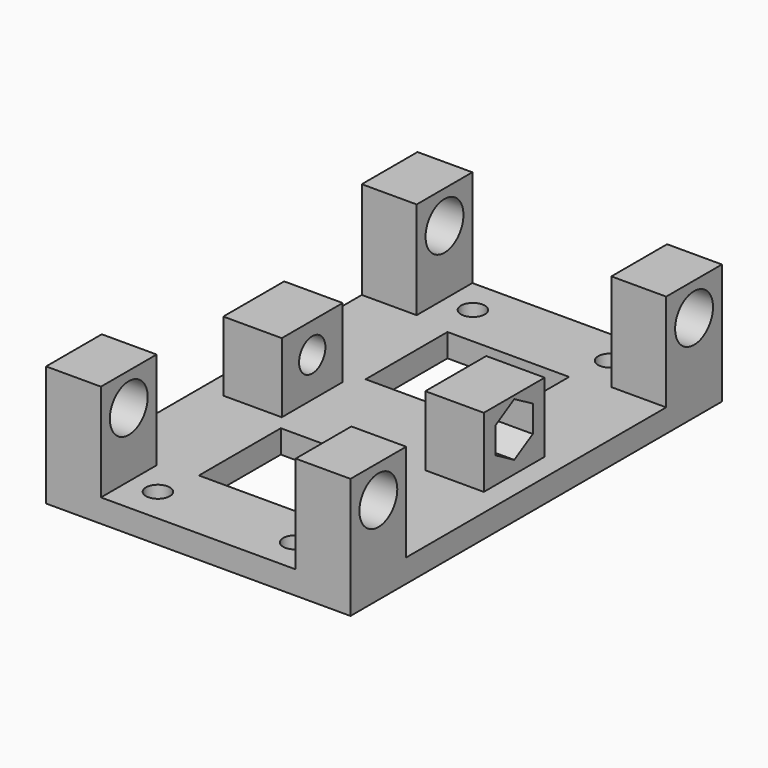
from build123d import *

# Parameters (mm, degrees)
F0_W      = 83.264
F0_H      = 127
F1_DEPTH  = 6.35
F2_W      = 15
F2_H      = 19.05
F3_DEPTH  = 26.67
F5_D      = 12.954
F7_D      = 6.528
F8_W      = 16
F8_H      = 20.828
F9_DEPTH  = 19.05
F11_DEPTH = 10
F13_DEPTH = 10
F15_D     = 9
F16_W     = 33.264
F16_H     = 28
F17_DEPTH = 6.351


# Not quite as in the source:
# - a feature names something its author has since deleted; it is built from what else it names


with BuildPart() as f1:
    # F0 (on Top) → F1 (new body)
    with BuildSketch(Plane.XY):
        with Locations((-3.6434741511, 1.1941809207)):
            Rectangle(F0_W, F0_H)
    extrude(amount=F1_DEPTH)

    # F2 (on face) → F3 (join)
    with BuildSketch(Plane.XY.offset(6.35)):
        with Locations((-37.7754741511, 55.1691809207)):
            Rectangle(F2_W, F2_H)
        with Locations((30.4885258489, 55.1691809207)):
            Rectangle(F2_W, F2_H)
        with Locations((30.4885258489, -52.7808190793)):
            Rectangle(F2_W, F2_H)
        with Locations((-37.7754741511, -52.7808190793)):
            Rectangle(F2_W, F2_H)
    extrude(amount=F3_DEPTH)

    # F5 (through all)
    with Locations(Plane(origin=(-45.2754741511, 0, 0), x_dir=(0, -1, 0), z_dir=(-1, 0, 0))):
        with Locations((-55.1691809207, 24.006), (52.7808190793, 24.006)):
            Hole(F5_D / 2)

    # F7 (through all)
    with Locations(Plane.XY.offset(6.35)):
        with Locations((-22.3994741511, 55.0421809207), (15.1125258489, 55.0421809207), (-22.3994741511, -52.6538190793), (15.1125258489, -52.6538190793)):
            Hole(F7_D / 2)

    # F8 (on face) → F9 (join)
    with BuildSketch(Plane.XY.offset(6.35)):
        with Locations((-31.2754741511, 1.1941809207)):
            Rectangle(F8_W, F8_H)
        with Locations((23.9885258489, 1.1941809207)):
            Rectangle(F8_W, F8_H)
    extrude(amount=F9_DEPTH)

    # F10 (on face) → F11 (cut)
    with BuildSketch(Plane(origin=(-39.2754741511, 0, 0), x_dir=(0, -1, 0), z_dir=(-1, 0, 0))):
        Polygon((5.1458190793, 13.4845992933), (5.1458190793, 20.8054007067), (-1.1941809207, 24.4658014133), (-7.5341809207, 20.8054007067), (-7.5341809207, 13.4845992933), (-1.1941809207, 9.8241985867), align=None)
    extrude(amount=-F11_DEPTH, mode=Mode.SUBTRACT)

    # F12 (on face) → F13 (cut)
    with BuildSketch(Plane.YZ.offset(31.9885258489)):
        Polygon((7.5341809207, 13.4845992933), (7.5341809207, 20.8054007067), (1.1941809207, 24.4658014133), (-5.1458190793, 20.8054007067), (-5.1458190793, 13.4845992933), (1.1941809207, 9.8241985867), align=None)
    extrude(amount=-F13_DEPTH, mode=Mode.SUBTRACT)

    # F15 (through all)
    with Locations(Plane(origin=(-29.2754741511, 0, 0), x_dir=(0, -1, 0), z_dir=(-1, 0, 0))):
        with Locations((-1.1941809207, 17.1448014133)):
            Hole(F15_D / 2)

    # F16 (on face) → F17 (cut, through all)
    with BuildSketch(Plane.XY.offset(6.35)):
        with Locations((-3.6434741511, 29.6941809207)):
            Rectangle(F16_W, F16_H)
        with Locations((-3.6434741511, -27.3058190793)):
            Rectangle(F16_W, F16_H)
    extrude(amount=-F17_DEPTH, mode=Mode.SUBTRACT)


solid = f1.part
